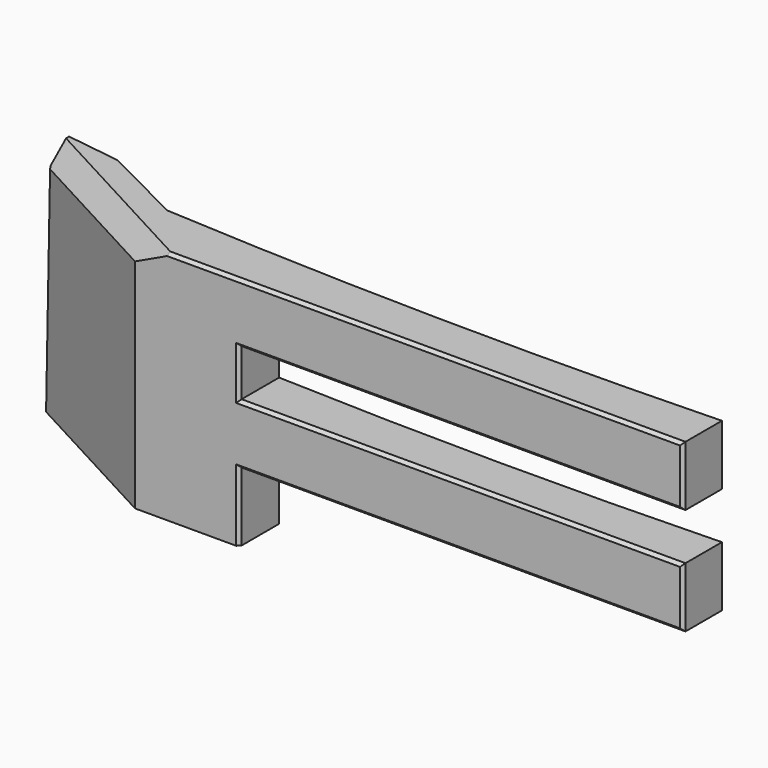
from build123d import *

# Parameters (mm, degrees)
F1_DEPTH     = 44.45
F4_DEPTH     = 98.5780825813
F5_SIZE      = 7.62
F6_T1_DEPTH  = 219.6945102582
F6_T3_DEPTH  = 31.6780747894
F6_T5_DEPTH  = 188.9400373947
F6_T7_DEPTH  = 31.6780747894
F6_T9_DEPTH  = 31.993119976
F6_T11_DEPTH = 19.558
F6_T13_DEPTH = 95.0320985588
F6_T19_DEPTH = 188.9400373947
F6_T23_DEPTH = 22.8240373947
F6_T30_DEPTH = 22.8240373947
F6_T34_DEPTH = 188.9400373947
F6_T41_DEPTH = 31.993119976
F6_T45_DEPTH = 188.9400373947
F7_T         = 3.81
F7_T3_DEPTH  = 9.8197045255
F7_T5_DEPTH  = 50.8
F7_T7_DEPTH  = 9.8197045256
F7_T9_DEPTH  = 9.8197045255
F8_R         = 4.0894
F8_R_2       = 1.8415
F9_DEPTH     = 40.64
F10_DEPTH    = 127


# Not quite as in the source:
# - a fillet or chamfer that OpenCascade refuses, or shapes differently, is made with other operations: its cross-section is extruded or revolved along the edge and cut away or added
# - a shell that OpenCascade refuses in one call is made with other operations: the cavity is built on its own and cut out


with BuildPart() as f1:
    # F0 (on Front) → F1 (new body)
    with BuildSketch(Plane.XZ):
        Polygon((-27.6737742102, 28.612719938), (-93.7137742102, 28.612719938), (-96.8887742102, -69.9643626433), (-17.5137742102, -69.9643626433), (12.7122257898, -69.9643626433), (12.7122257898, -41.237280062), (198.3862257898, -41.237280062), (198.3862257898, -16.091280062), (12.7122257898, -16.091280062), (12.7122257898, 3.466719938), (198.3862257898, 3.466719938), (198.3862257898, 28.612719938), align=None)
    extrude(amount=F1_DEPTH)

    # F2 (on face) → F4 (cut, through all)
    with BuildSketch(Plane(origin=(0, 0, -69.9643626433), x_dir=(1, 0, 0), z_dir=(0, 0, -1))):
        Polygon((-96.8887742102, 44.45), (-96.8887742102, 8.89), (-30.8487742102, 44.45), align=None)
    extrude(amount=-F4_DEPTH, mode=Mode.SUBTRACT)

    # F5
    f5_edges = [f1.edges().sort_by_distance(p)[0] for p in [
        (-62.281274, -27.524808, 28.61272),
    ]]
    chamfer(f5_edges, length=F5_SIZE)

    # F6: chamfer of 1.27 on 9 edges, made by hand

    # F6_s2 → F6_t1 (cut)
    with BuildSketch(Plane.YZ.offset(-18.0422470736)):
        Polygon((-43.18, 28.612719938), (-44.45, 27.342719938), (-44.45, 28.612719938), align=None)
    extrude(amount=F6_T1_DEPTH, mode=Mode.SUBTRACT)

    # F6_s4 → F6_t3 (cut)
    with BuildSketch(Plane.XY.offset(0.2006825433)):
        Polygon((197.1162257898, -44.45), (198.3862257898, -43.18), (198.3862257898, -44.45), align=None)
    extrude(amount=F6_T3_DEPTH, mode=Mode.SUBTRACT)

    # F6_s6 → F6_t5 (cut)
    with BuildSketch(Plane.YZ.offset(12.7122257898)):
        Polygon((-44.45, 4.736719938), (-43.18, 3.466719938), (-44.45, 3.466719938), align=None)
        Polygon((-44.45, -17.361280062), (-43.18, -16.091280062), (-44.45, -16.091280062), align=None)
        Polygon((-44.45, -39.967280062), (-43.18, -41.237280062), (-44.45, -41.237280062), align=None)
    extrude(amount=F6_T5_DEPTH, mode=Mode.SUBTRACT)

    # F6_s8 → F6_t7 (cut)
    with BuildSketch(Plane.XY.offset(-44.5033174567)):
        Polygon((197.1162257898, -44.45), (198.3862257898, -43.18), (198.3862257898, -44.45), align=None)
    extrude(amount=F6_T7_DEPTH, mode=Mode.SUBTRACT)

    # F6_s10 → F6_t9 (cut)
    with BuildSketch(Plane.XY.offset(-73.230400038)):
        Polygon((11.4422257898, -44.45), (12.7122257898, -43.18), (12.7122257898, -44.45), align=None)
    extrude(amount=F6_T9_DEPTH, mode=Mode.SUBTRACT)

    # F6_s12 → F6_t11 (cut)
    with BuildSketch(Plane.XY.offset(-16.091280062)):
        Polygon((11.4422257898, -44.45), (12.7122257898, -43.18), (12.7122257898, -44.45), align=None)
    extrude(amount=F6_T11_DEPTH, mode=Mode.SUBTRACT)

    # F6_s14 → F6_t13 (cut)
    with BuildSketch(Plane(origin=(-2.4104397516, 1.297929097, -74.8390924249), x_dir=(0.474099823, 0.8804710999, 0), z_dir=(0.0321867693, -0.0173313373, 0.9993315949))):
        Polygon((-53.0941334984, 78.8407390233), (-53.7623387855, 77.722372749), (-53.7623387855, 78.4811766705), align=None)
    extrude(amount=F6_T13_DEPTH, mode=Mode.SUBTRACT)


with BuildPart() as f6_tool17:
    # F6_s18 → F6_t19 (new body)
    with BuildSketch(Plane.YZ.offset(9.4461883951)):
        Polygon((-44.45, 4.736719938), (-43.18, 3.466719938), (-44.45, 3.466719938), align=None)
    extrude(amount=F6_T19_DEPTH)

    split(bisect_by=Plane.YZ.offset(12.7122257898), keep=Keep.BOTTOM)


with BuildPart() as f6_tool21:
    # F6_s22 → F6_t23 (new body)
    with BuildSketch(Plane.XY.offset(-16.091280062)):
        Polygon((11.4422257898, -44.45), (12.7122257898, -43.18), (12.7122257898, -44.45), align=None)
    extrude(amount=F6_T23_DEPTH)

    split(bisect_by=Plane.XY.offset(3.466719938), keep=Keep.TOP)


with BuildPart() as f6_tool17_1:
    add(f6_tool17.part)

    # F6_t25: intersect F6_tool21
    add(f6_tool21.part, mode=Mode.INTERSECT)


with BuildPart() as f1_1:
    add(f1.part)

    # F6_t15: cut F6_tool17
    add(f6_tool17_1.part, mode=Mode.SUBTRACT)


with BuildPart() as f6_tool28:
    # F6_s29 → F6_t30 (new body)
    with BuildSketch(Plane.XY.offset(-19.3573174567)):
        Polygon((11.4422257898, -44.45), (12.7122257898, -43.18), (12.7122257898, -44.45), align=None)
    extrude(amount=F6_T30_DEPTH)

    split(bisect_by=Plane.XY.offset(-16.091280062), keep=Keep.BOTTOM)


with BuildPart() as f6_tool32:
    # F6_s33 → F6_t34 (new body)
    with BuildSketch(Plane.YZ.offset(198.3862257898)):
        Polygon((-44.45, -17.361280062), (-43.18, -16.091280062), (-44.45, -16.091280062), align=None)
    extrude(amount=-F6_T34_DEPTH)

    split(bisect_by=Plane.YZ.offset(12.7122257898), keep=Keep.BOTTOM)


with BuildPart() as f6_tool28_1:
    add(f6_tool28.part)

    # F6_t36: intersect F6_tool32
    add(f6_tool32.part, mode=Mode.INTERSECT)


with BuildPart() as f1_2:
    add(f1_1.part)

    # F6_t26: cut F6_tool28
    add(f6_tool28_1.part, mode=Mode.SUBTRACT)


with BuildPart() as f6_tool39:
    # F6_s40 → F6_t41 (new body)
    with BuildSketch(Plane.XY.offset(-69.9643626433)):
        Polygon((11.4422257898, -44.45), (12.7122257898, -43.18), (12.7122257898, -44.45), align=None)
    extrude(amount=F6_T41_DEPTH)

    split(bisect_by=Plane.XY.offset(-41.237280062), keep=Keep.TOP)


with BuildPart() as f6_tool43:
    # F6_s44 → F6_t45 (new body)
    with BuildSketch(Plane.YZ.offset(9.4461883951)):
        Polygon((-44.45, -39.967280062), (-43.18, -41.237280062), (-44.45, -41.237280062), align=None)
    extrude(amount=F6_T45_DEPTH)

    split(bisect_by=Plane.YZ.offset(12.7122257898), keep=Keep.BOTTOM)


with BuildPart() as f6_tool39_1:
    add(f6_tool39.part)

    # F6_t47: intersect F6_tool43
    add(f6_tool43.part, mode=Mode.INTERSECT)


with BuildPart() as f1_3:
    add(f1_2.part)

    # F6_t37: cut F6_tool39
    add(f6_tool39_1.part, mode=Mode.SUBTRACT)

    # F7: shell of thickness 3.81, made by hand


with BuildPart() as f7_core1:
    # F7_t2: copy of F1
    add(f1_3.part)

    # the walls: a layer under each face that stays
    f7_faces = [f7_core1.faces().sort_by_distance(p)[0] for p in [
        (52.3362257898, -21.59, 28.612719938),
        (-95.3012742102, -4.8600664948, -20.6758213526),
        (-95.0796094442, -9.4847066882, -24.1721603779),
        (-63.5344983168, -26.8499947118, -24.4858213526),
        (83.1337257898, -44.45, -21.3108213526),
        (197.7512257898, -43.815, 16.039719938),
        (104.9142257898, -43.815, 4.101719938),
        (105.5492257898, -21.59, 3.466719938),
        (12.7122257898, -21.59, -6.312280062),
        (105.5492257898, -21.59, -16.091280062),
        (198.3862257898, -21.59, -28.664280062),
        (105.5492257898, -21.59, -41.237280062),
        (12.7122257898, -21.59, -55.6008213526),
        (12.0772257898, -43.815, -6.312280062),
        (104.9142257898, -43.815, -16.726280062),
        (197.7512257898, -43.815, -28.664280062),
        (104.9142257898, -43.815, -40.602280062),
        (12.0772257898, -43.815, -54.9658213526),
        (-42.0882742102, -22.225, -69.9643626433),
        (198.3862257898, -21.59, 16.039719938),
        (90.4656276778, -43.815, 27.977719938),
        (-57.0896392603, -25.9930745223, 24.802719938),
    ]]
    thicken(f7_faces, amount=-F7_T, mode=Mode.SUBTRACT)

    # F7_s4 → F7_t3 (cut)
    with BuildSketch(Plane(origin=(-9.1117935238, -9.1117935238, 9.1117935238), x_dir=(0.7071067812, -0.7071067812, 0), z_dir=(-0.5773502692, -0.5773502692, 0.5773502692))):
        Polygon((39.5789218716, -9.640847327), (37.6167718716, -6.3082949707), (35.7117718716, -7.4081472335), (35.7117718716, -9.6078517591), align=None)
    extrude(amount=F7_T3_DEPTH, mode=Mode.SUBTRACT)

    # F7_s6 → F7_t5 (cut)
    with BuildSketch(Plane.XZ.offset(-3.81)):
        Polygon((12.7503257898, 3.428619938), (12.7122257898, 7.276719938), (8.9022257898, 7.276719938), (8.9022257898, 3.466719938), align=None)
        Polygon((12.7503257898, -16.053180062), (8.9022257898, -16.091280062), (8.9022257898, -19.901280062), (12.7122257898, -19.901280062), align=None)
        Polygon((12.7503257898, -41.275380062), (12.7122257898, -37.427280062), (8.9022257898, -37.427280062), (8.9022257898, -41.237280062), align=None)
    extrude(amount=F7_T5_DEPTH, mode=Mode.SUBTRACT)

    # F7_s8 → F7_t7 (cut)
    with BuildSketch(Plane(origin=(-13.3199802318, -13.3199802318, -13.3199802318), x_dir=(0.7071067812, -0.7071067812, 0), z_dir=(-0.5773502692, -0.5773502692, -0.5773502692))):
        Polygon((39.5789218716, -0.6670628499), (35.7117718716, -0.7000584178), (35.7117718716, -2.8997629434), (37.6167718716, -3.9996152062), align=None)
    extrude(amount=F7_T7_DEPTH, mode=Mode.SUBTRACT)

    # F7_s10 → F7_t9 (cut)
    with BuildSketch(Plane(origin=(0.1201307583, 0.1201307583, -0.1201307583), x_dir=(-0.7071067812, 0.7071067812, 0), z_dir=(0.5773502692, 0.5773502692, -0.5773502692))):
        Polygon((-39.5789218716, -46.1415104808), (-37.6167718716, -42.8089581245), (-35.7117718716, -43.9088103873), (-35.7117718716, -46.1085149129), align=None)
    extrude(amount=F7_T9_DEPTH, mode=Mode.SUBTRACT)


with BuildPart() as f1_4:
    add(f1_3.part)

    # what is left inside the walls is the cavity
    f7_cavity = [f7_core1.part.solids().sort_by_distance(p)[0] for p in [
        (50.81107, -0.0381, -35.835335),
    ]]
    add(f7_cavity, mode=Mode.SUBTRACT)

    # F8 (on face) → F9 (join, through all)
    with BuildSketch(Plane(origin=(0, -40.64, 0), x_dir=(-1, 0, 0), z_dir=(0, 1, 0))):
        with Locations((-167.5252257898, 14.642719938)):
            Circle(F8_R)
        with Locations((-167.5252257898, 14.642719938)):
            Circle(F8_R_2, mode=Mode.SUBTRACT)
        with Locations((-109.7656257898, 14.642719938)):
            Circle(F8_R)
        with Locations((-109.7656257898, 14.642719938)):
            Circle(F8_R_2, mode=Mode.SUBTRACT)
        with Locations((9.3857742102, -44.920280062)):
            Circle(F8_R)
        with Locations((9.3857742102, -44.920280062)):
            Circle(F8_R_2, mode=Mode.SUBTRACT)
        with Locations((9.3857742102, 4.609719938)):
            Circle(F8_R)
        with Locations((9.3857742102, 4.609719938)):
            Circle(F8_R_2, mode=Mode.SUBTRACT)
    extrude(amount=F9_DEPTH)

    # F3 (on face) → F10 (cut, symmetric)
    with BuildSketch(Plane(origin=(0, 0, -41.237280062), x_dir=(1, 0, 0), z_dir=(0, 0, -1))):
        with BuildLine():
            Line((-70.9720987785, 3.4942372568), (-96.1306024302, 0))
            Line((-96.1306024302, 0), (198.3862257898, 0))
            Line((198.3862257898, 0), (198.3862257898, 24.13))
            ThreePointArc((198.3862257898, 24.13), (81.1301273633, 25.39290124), (-36.0551004282, 21.1255923438))
            Line((-36.0551004282, 21.1255923438), (-70.9720987785, 3.4942372568))
        make_face()
    extrude(amount=F10_DEPTH, both=True, mode=Mode.SUBTRACT)


solid = f1_4.part
